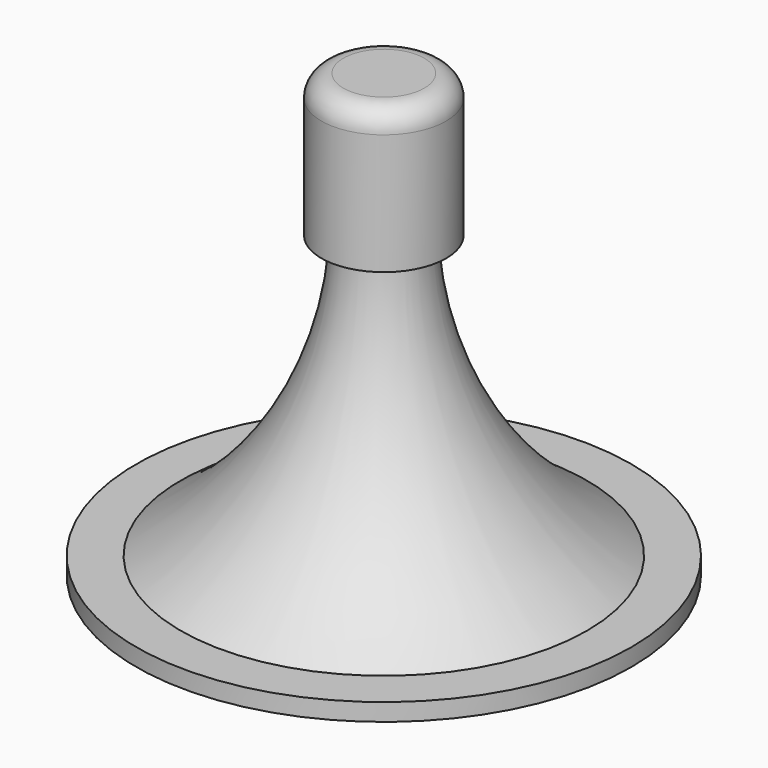
from build123d import *

# Parameters (mm, degrees)
F2_R    = 1.19999
F5_R    = 3
F6_SIZE = 1.5
F7_SIZE = 2.39999
F8_R    = 1


# Not quite as in the source:
# - a fillet or chamfer is up to 0.001 mm smaller than in the source, because OpenCascade refuses the exact size
# - a feature names something its author has since deleted; it is built from what else it names


with BuildPart() as f1:
    # F0 (on Front) → F1 (revolve)
    with BuildSketch(Plane.XZ):
        with BuildLine():
            Line((24.4990454972, 2.4), (24.4990454972, 0))
            Line((24.4990454972, 0), (33.9990454972, 0))
            Line((33.9990454972, 0), (33.9990454972, 2.4))
            Line((33.9990454972, 2.4), (27.8990454972, 2.4))
            ThreePointArc((27.8990454972, 2.4), (11.680396645, 19.9385185195), (5.7987742726, 43.0912876998))
            Line((5.7987742726, 43.0912876998), (5.7987742726, 44.2659604814))
            Line((5.7987742726, 44.2659604814), (5.7987742726, 58.0912876998))
            Line((5.7987742726, 58.0912876998), (3.3987742726, 58.0912876998))
            Line((3.3987742726, 58.0912876998), (3.3987742726, 43.0912876998))
            ThreePointArc((3.3987742726, 43.0912876998), (8.9875250867, 20.1729416621), (24.4990454972, 2.4))
        make_face()
        with BuildLine():
            Line((5.7987742726, 44.2659604814), (5.7987742726, 43.0912876998))
            ThreePointArc((5.7987742726, 43.0912876998), (6.1703214686, 43.6786240906), (5.7987742726, 44.2659604814))
        make_face()
    revolve(axis=Axis((0, 0, 21.5), (0, 0, 1)))

    # F2 (radius 1.2 in the source; OpenCascade refuses exactly that, so slightly less here)
    f2_edges = [f1.edges().sort_by_distance(p)[0] for p in [
        (-5.798774, 0, 58.091288),
        (-3.398774, 0, 58.091288),
    ]]
    fillet(f2_edges, radius=F2_R)

    # F7 (size 2.4 in the source; OpenCascade refuses exactly that, so slightly less here)
    f7_edges = [f1.edges().sort_by_distance(p)[0] for p in [
        (-24.499045, 0, 0),
    ]]
    chamfer(f7_edges, length=F7_SIZE)


with BuildPart() as f4:
    # F3 (on Front) → F4 (revolve)
    with BuildSketch(Plane.XZ):
        with BuildLine():
            Line((3.1987742726, 58.2966972564), (6.0987742726, 58.2966972564))
            Line((6.0987742726, 58.2966972564), (6.0987742726, 44.7102859616))
            ThreePointArc((6.0987742726, 44.7102859616), (6.4848899514, 43.868804239), (6.0987742726, 43.0273225163))
            Line((6.0987742726, 43.0273225163), (6.1624427434, 41.1088836943))
            Line((6.1624427434, 41.1088836943), (8.5624427434, 41.1088836943))
            Line((8.5624427434, 41.1088836943), (8.5624427434, 60.6966972564))
            Line((8.5624427434, 60.6966972564), (0, 60.6966972564))
            Line((0, 60.6966972564), (0, 54.5966972564))
            Line((0, 54.5966972564), (3.1987742726, 54.5966972564))
            Line((3.1987742726, 54.5966972564), (3.1987742726, 58.2966972564))
        make_face()
    revolve(axis=Axis((0, 0, 21.5), (0, 0, 1)))

    # F5
    f5_edges = [f4.edges().sort_by_distance(p)[0] for p in [
        (-8.562443, 0, 60.696697),
    ]]
    fillet(f5_edges, radius=F5_R)

    # F6
    f6_edges = [f4.edges().sort_by_distance(p)[0] for p in [
        (-3.198774, 0, 54.596697),
    ]]
    chamfer(f6_edges, length=F6_SIZE)

    # F8
    f8_edges = [f4.edges().sort_by_distance(p)[0] for p in [
        (-6.098774, 0, 58.296697),
    ]]
    fillet(f8_edges, radius=F8_R)


solid = Compound([f1.part, f4.part])
